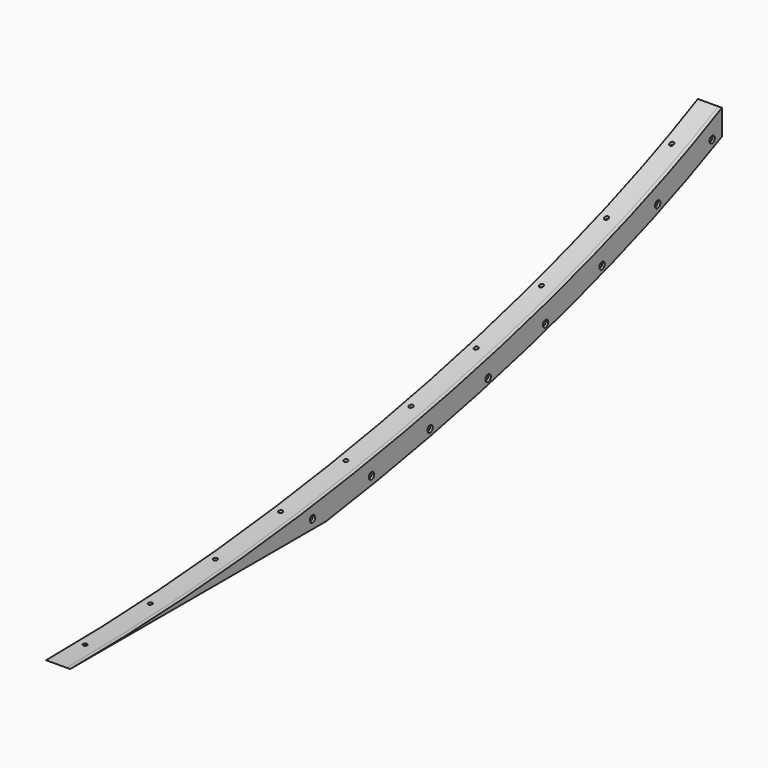
from build123d import *

# Parameters (mm, degrees)
F1_DEPTH      = 4.5
F1_DEPTH_BACK = 25
F2_DEPTH      = 4.5
F3_DEPTH      = 1.5
F4_R          = 2.5
F5_DEPTH      = 150
F6_R          = 4.1800646045
F7_DEPTH      = 12.5


# Not quite as in the source:
# - the dataset's text gives a spline's control points without its knots; the knots are read off the source's solid


with BuildPart() as f1:
    # F0 (on Right) → F1 (new body, two sides)
    with BuildSketch(Plane.YZ) as f1_sk:
        with BuildLine():
            add(Edge.make_bspline(
                [(-542.9529296271, -39.9508323044), (-188.0693441655, -39.9508323044), (204.5968802247, 34.2876766354), (457.0470703729, 160.0491676956)],
                knots=[0, 0, 0, 0, 1019.8039027186, 1019.8039027186, 1019.8039027186, 1019.8039027186], degree=3))
            Line((-542.9529296271, -39.9508323044), (-417.3127151335, -39.9508323044))
            add(Edge.make_bspline(
                [(-417.3127151335, -39.9508323044), (-369.1001563129, -37.6799090107), (-229.605831227, -27.4883990926), (-0.7659143619, 6.0089411279), (250.4802761754, 69.14721948), (394.0857076642, 125.4398419701), (457.047070373, 156.6986558412)],
                knots=[0.116693999, 0.116693999, 0.116693999, 0.116693999, 0.25, 0.5, 0.75, 0.9982402372, 0.9982402372, 0.9982402372, 0.9982402372], degree=3))
            Line((457.0470703729, 156.6986558412), (457.0470703729, 160.0491676956))
        make_face()
    extrude(amount=F1_DEPTH)
    extrude(f1_sk.sketch, amount=-F1_DEPTH_BACK)

    # F0 (on Right) → F2 (join, symmetric)
    with BuildSketch(Plane.YZ):
        with BuildLine():
            add(Edge.make_bspline(
                [(-417.3127151335, -39.9508323044), (-369.1001563129, -37.6799090107), (-229.605831227, -27.4883990926), (-0.7659143619, 6.0089411279), (250.4802761754, 69.14721948), (394.0857076642, 125.4398419701), (457.047070373, 156.6986558412)],
                knots=[0.116693999, 0.116693999, 0.116693999, 0.116693999, 0.25, 0.5, 0.75, 0.9982402372, 0.9982402372, 0.9982402372, 0.9982402372], degree=3))
            Line((-417.3127151335, -39.9508323044), (-149.937543661, -39.9508323044))
            add(Edge.make_bspline(
                [(-149.937543661, -39.9508323044), (-98.996798705, -32.7943859429), (-3.7016307054, -16.778446645), (131.246444394, 13.3933570474), (254.1058325956, 48.1234806847), (363.3774188375, 86.6936370443), (428.3490574687, 114.995507991), (457.0470703729, 128.861665731)],
                knots=[0.3594995159, 0.3594995159, 0.3594995159, 0.3594995159, 0.5, 0.625, 0.75, 0.875, 0.9840561675, 0.9840561675, 0.9840561675, 0.9840561675], degree=3))
            Line((457.0470703729, 128.861665731), (457.0470703729, 156.6986558412))
        make_face()
    extrude(amount=F2_DEPTH, both=True)

    # F0 (on Right) → F3 (cut, symmetric)
    with BuildSketch(Plane.YZ):
        with BuildLine():
            add(Edge.make_bspline(
                [(-417.3127151335, -39.9508323044), (-369.1001563129, -37.6799090107), (-229.605831227, -27.4883990926), (-0.7659143619, 6.0089411279), (250.4802761754, 69.14721948), (394.0857076642, 125.4398419701), (457.047070373, 156.6986558412)],
                knots=[0.116693999, 0.116693999, 0.116693999, 0.116693999, 0.25, 0.5, 0.75, 0.9982402372, 0.9982402372, 0.9982402372, 0.9982402372], degree=3))
            Line((-417.3127151335, -39.9508323044), (-149.937543661, -39.9508323044))
            add(Edge.make_bspline(
                [(-149.937543661, -39.9508323044), (-98.996798705, -32.7943859429), (-3.7016307054, -16.778446645), (131.246444394, 13.3933570474), (254.1058325956, 48.1234806847), (363.3774188375, 86.6936370443), (428.3490574687, 114.995507991), (457.0470703729, 128.861665731)],
                knots=[0.3594995159, 0.3594995159, 0.3594995159, 0.3594995159, 0.5, 0.625, 0.75, 0.875, 0.9840561675, 0.9840561675, 0.9840561675, 0.9840561675], degree=3))
            Line((457.0470703729, 128.861665731), (457.0470703729, 156.6986558412))
        make_face()
    extrude(amount=F3_DEPTH, both=True, mode=Mode.SUBTRACT)

    # F4 (on Top) → F5 (cut, symmetric)
    with BuildSketch(Plane.XY):
        with Locations((-15.5, -494.9529296271)):
            Circle(F4_R)
        with Locations((-15.5, -394.9529296271)):
            Circle(F4_R)
        with Locations((-15.5, -294.9529296271)):
            Circle(F4_R)
        with Locations((-15.5, -194.9529296271)):
            Circle(F4_R)
        with Locations((-15.5, -94.9529296271)):
            Circle(F4_R)
        with Locations((-15.5, 5.0470703729)):
            Circle(F4_R)
        with Locations((-15.5, 105.0470703729)):
            Circle(F4_R)
        with Locations((-15.5, 205.0470703729)):
            Circle(F4_R)
        with Locations((-15.5, 305.0470703729)):
            Circle(F4_R)
        with Locations((-15.5, 405.0470703729)):
            Circle(F4_R)
        with Locations((-45.5, -494.9529296271)):
            Circle(F4_R)
        with Locations((-45.5, -394.9529296271)):
            Circle(F4_R)
        with Locations((-45.5, -294.9529296271)):
            Circle(F4_R)
        with Locations((-45.5, -194.9529296271)):
            Circle(F4_R)
        with Locations((-45.5, -94.9529296271)):
            Circle(F4_R)
        with Locations((-45.5, 5.0470703729)):
            Circle(F4_R)
        with Locations((-45.5, 105.0470703729)):
            Circle(F4_R)
        with Locations((-45.5, 205.0470703729)):
            Circle(F4_R)
        with Locations((-45.5, 305.0470703729)):
            Circle(F4_R)
        with Locations((-45.5, 405.0470703729)):
            Circle(F4_R)
    extrude(amount=F5_DEPTH, both=True, mode=Mode.SUBTRACT)

    # F6 (on Right) → F7 (cut, symmetric)
    with BuildSketch(Plane.YZ):
        with Locations((442.0470703729, 131.861665731)):
            Circle(F6_R)
        with Locations((358.44841201, 95.9379511725)):
            Circle(F6_R)
        with Locations((273.163023997, 64.2259417875)):
            Circle(F6_R)
        with Locations((186.4029392463, 36.8044786279)):
            Circle(F6_R)
        with Locations((98.3838569987, 13.7417357717)):
            Circle(F6_R)
        with Locations((9.3246065611, -4.9049491686)):
            Circle(F6_R)
        with Locations((-80.5533967375, -19.0892175961)):
            Circle(F6_R)
        with Locations((-171.0267020195, -28.7758051847)):
            Circle(F6_R)
    extrude(amount=F7_DEPTH, both=True, mode=Mode.SUBTRACT)


solid = f1.part
